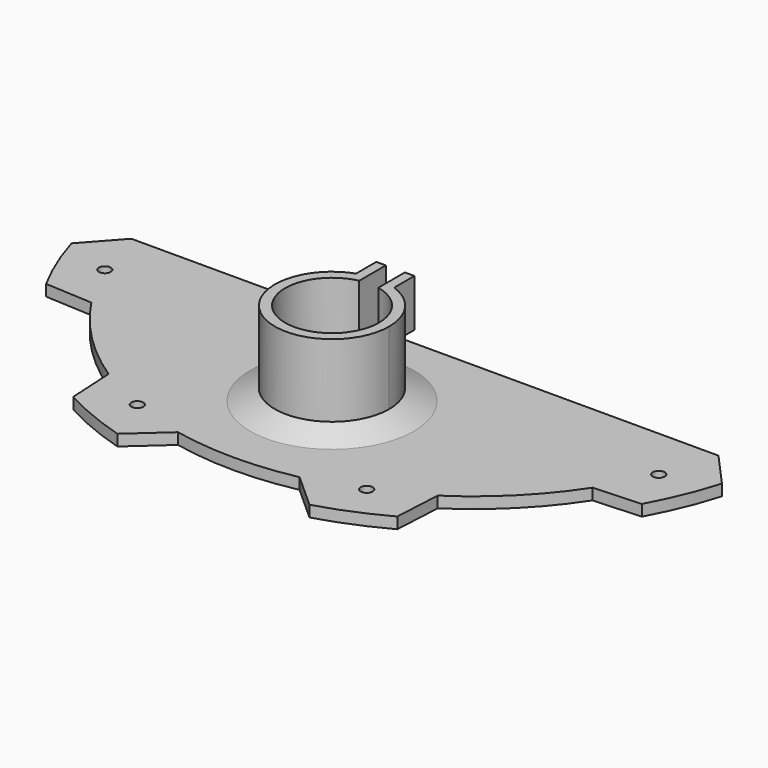
from build123d import *

# Parameters (mm, degrees)
F0_R     = 1.5875
F0_R_2   = 22.225
F1_DEPTH = 2.9972
F2_DEPTH = 25.4
F3_DEPTH = 25.4
F4_DEPTH = 12.7
F5_DEPTH = 2.9972
F6_DEPTH = 5.9944


# Not quite as in the source:
# - a fillet or chamfer that OpenCascade refuses, or shapes differently, is made with other operations: its cross-section is extruded or revolved along the edge and cut away or added


with BuildPart() as f1:
    # F0 (on Top) → F1 (new body)
    with BuildSketch(Plane.XY):
        with BuildLine():
            Line((-78.3343552322, -16.2264228234), (-86.7801633577, -25.6357348999))
            ThreePointArc((-86.7801633577, -25.6357348999), (-83.5995491981, -34.6280670861), (-79.4900439712, -43.2356399943))
            Line((-79.4900439712, -43.2356399943), (-66.8645673974, -43.9169401718))
            ThreePointArc((-66.8645673974, -43.9169401718), (-56.5666333066, -56.5666333066), (-43.9169401718, -66.8645673974))
            Line((-43.9169401718, -66.8645673974), (-43.2356399943, -79.4900439712))
            ThreePointArc((-43.2356399943, -79.4900439712), (-34.6280670861, -83.5995491981), (-25.6357348999, -86.7801633577))
            Line((-25.6357348999, -86.7801633577), (-16.2264228234, -78.3343552322))
            ThreePointArc((-16.2264228234, -78.3343552322), (0, -79.9973), (16.2264228234, -78.3343552322))
            Line((16.2264228234, -78.3343552322), (25.6357348999, -86.7801633577))
            ThreePointArc((25.6357348999, -86.7801633577), (34.6280670861, -83.5995491981), (43.2356399943, -79.4900439712))
            Line((43.2356399943, -79.4900439712), (43.9169401718, -66.8645673974))
            ThreePointArc((43.9169401718, -66.8645673974), (56.5666333066, -56.5666333066), (66.8645673974, -43.9169401718))
            Line((66.8645673974, -43.9169401718), (79.4900439712, -43.2356399943))
            ThreePointArc((79.4900439712, -43.2356399943), (83.5995491981, -34.6280670861), (86.7801633577, -25.6357348999))
            Line((86.7801633577, -25.6357348999), (78.3343552322, -16.2264228234))
            Line((78.3343552322, -16.2264228234), (-78.3343552322, -16.2264228234))
        make_face()
        with Locations((-30.6136413439, -73.9078681262)):
            Circle(F0_R, mode=Mode.SUBTRACT)
        with Locations((30.6136413439, -73.9078681262)):
            Circle(F0_R, mode=Mode.SUBTRACT)
        with Locations((0, -47.218952328)):
            Circle(F0_R_2, mode=Mode.SUBTRACT)
        with Locations((-73.9078681262, -30.6136413439)):
            Circle(F0_R, mode=Mode.SUBTRACT)
        with Locations((73.9078681262, -30.6136413439)):
            Circle(F0_R, mode=Mode.SUBTRACT)
        with Locations((0, -47.218952328)):
            Circle(F0_R_2)
        with BuildLine():
            ThreePointArc((5.08, -32.8505425343), (12.4434078933, -38.4201342255), (15.24, -47.218952328))
            ThreePointArc((15.24, -47.218952328), (-8.7988181024, -59.6623602213), (-5.08, -32.8505425343))
            Line((-5.08, -32.8505425343), (-5.08, -26.0933935642))
            Line((-5.08, -26.0933935642), (-2.54, -26.0933935642))
            Line((-2.54, -26.0933935642), (-2.54, -32.1921096789))
            ThreePointArc((-2.54, -32.1921096789), (0, -31.978952328), (2.54, -32.1921096789))
            Line((2.54, -32.1921096789), (2.54, -26.0933935642))
            Line((2.54, -26.0933935642), (5.08, -26.0933935642))
            Line((5.08, -26.0933935642), (5.08, -32.8505425343))
        make_face(mode=Mode.SUBTRACT)
        with BuildLine():
            ThreePointArc((-5.08, -32.8505425343), (-8.7988181024, -59.6623602213), (15.24, -47.218952328))
            ThreePointArc((15.24, -47.218952328), (12.4434078933, -38.4201342255), (5.08, -32.8505425343))
            ThreePointArc((5.08, -32.8505425343), (3.8241970996, -32.466558741), (2.54, -32.1921096789))
            Line((2.54, -32.1921096789), (2.54, -34.9700344064))
            ThreePointArc((2.54, -34.9700344064), (9.7021059634, -39.3223245588), (12.5095, -47.218952328))
            ThreePointArc((12.5095, -47.218952328), (-7.8966277692, -56.9210582914), (-2.54, -34.9700344064))
            Line((-2.54, -34.9700344064), (-2.54, -32.1921096789))
            ThreePointArc((-2.54, -32.1921096789), (-3.8241970996, -32.466558741), (-5.08, -32.8505425343))
        make_face()
        with BuildLine():
            ThreePointArc((2.54, -32.1921096789), (3.8241970996, -32.466558741), (5.08, -32.8505425343))
            Line((5.08, -32.8505425343), (5.08, -26.0933935642))
            Line((5.08, -26.0933935642), (2.54, -26.0933935642))
            Line((2.54, -26.0933935642), (2.54, -32.1921096789))
        make_face()
        with BuildLine():
            Line((-5.08, -26.0933935642), (-5.08, -32.8505425343))
            ThreePointArc((-5.08, -32.8505425343), (-3.8241970996, -32.466558741), (-2.54, -32.1921096789))
            Line((-2.54, -32.1921096789), (-2.54, -26.0933935642))
            Line((-2.54, -26.0933935642), (-5.08, -26.0933935642))
        make_face()
        with BuildLine():
            Line((2.54, -34.9700344064), (2.54, -32.1921096789))
            ThreePointArc((2.54, -32.1921096789), (0, -31.978952328), (-2.54, -32.1921096789))
            Line((-2.54, -32.1921096789), (-2.54, -34.9700344064))
            ThreePointArc((-2.54, -34.9700344064), (0, -34.709452328), (2.54, -34.9700344064))
        make_face()
        with BuildLine():
            ThreePointArc((12.5095, -47.218952328), (9.7021059634, -39.3223245588), (2.54, -34.9700344064))
            ThreePointArc((2.54, -34.9700344064), (0, -34.709452328), (-2.54, -34.9700344064))
            ThreePointArc((-2.54, -34.9700344064), (-7.8966277692, -56.9210582914), (12.5095, -47.218952328))
        make_face()
    extrude(amount=F1_DEPTH)

    # F0 (on Top) → F2 (join)
    with BuildSketch(Plane.XY):
        with BuildLine():
            ThreePointArc((-5.08, -32.8505425343), (-8.7988181024, -59.6623602213), (15.24, -47.218952328))
            ThreePointArc((15.24, -47.218952328), (12.4434078933, -38.4201342255), (5.08, -32.8505425343))
            ThreePointArc((5.08, -32.8505425343), (3.8241970996, -32.466558741), (2.54, -32.1921096789))
            Line((2.54, -32.1921096789), (2.54, -34.9700344064))
            ThreePointArc((2.54, -34.9700344064), (9.7021059634, -39.3223245588), (12.5095, -47.218952328))
            ThreePointArc((12.5095, -47.218952328), (-7.8966277692, -56.9210582914), (-2.54, -34.9700344064))
            Line((-2.54, -34.9700344064), (-2.54, -32.1921096789))
            ThreePointArc((-2.54, -32.1921096789), (-3.8241970996, -32.466558741), (-5.08, -32.8505425343))
        make_face()
    extrude(amount=F2_DEPTH)

    # F0 (on Top) → F3 (join)
    with BuildSketch(Plane.XY):
        with BuildLine():
            ThreePointArc((-5.08, -32.8505425343), (-8.7988181024, -59.6623602213), (15.24, -47.218952328))
            ThreePointArc((15.24, -47.218952328), (12.4434078933, -38.4201342255), (5.08, -32.8505425343))
            ThreePointArc((5.08, -32.8505425343), (3.8241970996, -32.466558741), (2.54, -32.1921096789))
            Line((2.54, -32.1921096789), (2.54, -34.9700344064))
            ThreePointArc((2.54, -34.9700344064), (9.7021059634, -39.3223245588), (12.5095, -47.218952328))
            ThreePointArc((12.5095, -47.218952328), (-7.8966277692, -56.9210582914), (-2.54, -34.9700344064))
            Line((-2.54, -34.9700344064), (-2.54, -32.1921096789))
            ThreePointArc((-2.54, -32.1921096789), (-3.8241970996, -32.466558741), (-5.08, -32.8505425343))
        make_face()
        with BuildLine():
            ThreePointArc((2.54, -32.1921096789), (3.8241970996, -32.466558741), (5.08, -32.8505425343))
            Line((5.08, -32.8505425343), (5.08, -26.0933935642))
            Line((5.08, -26.0933935642), (2.54, -26.0933935642))
            Line((2.54, -26.0933935642), (2.54, -32.1921096789))
        make_face()
        with BuildLine():
            Line((-5.08, -26.0933935642), (-5.08, -32.8505425343))
            ThreePointArc((-5.08, -32.8505425343), (-3.8241970996, -32.466558741), (-2.54, -32.1921096789))
            Line((-2.54, -32.1921096789), (-2.54, -26.0933935642))
            Line((-2.54, -26.0933935642), (-5.08, -26.0933935642))
        make_face()
    extrude(amount=F3_DEPTH)

    # F0 (on Top) → F4 (cut)
    with BuildSketch(Plane.XY):
        with BuildLine():
            ThreePointArc((2.54, -32.1921096789), (3.8241970996, -32.466558741), (5.08, -32.8505425343))
            Line((5.08, -32.8505425343), (5.08, -26.0933935642))
            Line((5.08, -26.0933935642), (2.54, -26.0933935642))
            Line((2.54, -26.0933935642), (2.54, -32.1921096789))
        make_face()
        with BuildLine():
            Line((-5.08, -26.0933935642), (-5.08, -32.8505425343))
            ThreePointArc((-5.08, -32.8505425343), (-3.8241970996, -32.466558741), (-2.54, -32.1921096789))
            Line((-2.54, -32.1921096789), (-2.54, -26.0933935642))
            Line((-2.54, -26.0933935642), (-5.08, -26.0933935642))
        make_face()
    extrude(amount=F4_DEPTH, mode=Mode.SUBTRACT)

    # F0 (on Top) → F5 (join)
    with BuildSketch(Plane.XY):
        with BuildLine():
            ThreePointArc((2.54, -32.1921096789), (3.8241970996, -32.466558741), (5.08, -32.8505425343))
            Line((5.08, -32.8505425343), (5.08, -26.0933935642))
            Line((5.08, -26.0933935642), (2.54, -26.0933935642))
            Line((2.54, -26.0933935642), (2.54, -32.1921096789))
        make_face()
        with BuildLine():
            Line((-5.08, -26.0933935642), (-5.08, -32.8505425343))
            ThreePointArc((-5.08, -32.8505425343), (-3.8241970996, -32.466558741), (-2.54, -32.1921096789))
            Line((-2.54, -32.1921096789), (-2.54, -26.0933935642))
            Line((-2.54, -26.0933935642), (-5.08, -26.0933935642))
        make_face()
    extrude(amount=F5_DEPTH)

    # F0 (on Top) → F6 (join)
    with BuildSketch(Plane.XY):
        with Locations((0, -47.218952328)):
            Circle(F0_R_2)
        with BuildLine():
            ThreePointArc((5.08, -32.8505425343), (12.4434078933, -38.4201342255), (15.24, -47.218952328))
            ThreePointArc((15.24, -47.218952328), (-8.7988181024, -59.6623602213), (-5.08, -32.8505425343))
            Line((-5.08, -32.8505425343), (-5.08, -26.0933935642))
            Line((-5.08, -26.0933935642), (-2.54, -26.0933935642))
            Line((-2.54, -26.0933935642), (-2.54, -32.1921096789))
            ThreePointArc((-2.54, -32.1921096789), (0, -31.978952328), (2.54, -32.1921096789))
            Line((2.54, -32.1921096789), (2.54, -26.0933935642))
            Line((2.54, -26.0933935642), (5.08, -26.0933935642))
            Line((5.08, -26.0933935642), (5.08, -32.8505425343))
        make_face(mode=Mode.SUBTRACT)
        with BuildLine():
            ThreePointArc((2.54, -32.1921096789), (3.8241970996, -32.466558741), (5.08, -32.8505425343))
            Line((5.08, -32.8505425343), (5.08, -26.0933935642))
            Line((5.08, -26.0933935642), (2.54, -26.0933935642))
            Line((2.54, -26.0933935642), (2.54, -32.1921096789))
        make_face()
        with BuildLine():
            Line((-5.08, -26.0933935642), (-5.08, -32.8505425343))
            ThreePointArc((-5.08, -32.8505425343), (-3.8241970996, -32.466558741), (-2.54, -32.1921096789))
            Line((-2.54, -32.1921096789), (-2.54, -26.0933935642))
            Line((-2.54, -26.0933935642), (-5.08, -26.0933935642))
        make_face()
    extrude(amount=F6_DEPTH)

    # F7: chamfer of 6.858 x 3.1496 on 1 edges, made by hand


with BuildPart() as f7_tool2:
    # F7_s3 → F7_t4 (revolve)
    with BuildSketch(Plane.XZ.offset(47.218952328)):
        Polygon((22.225, 2.8448), (15.367, 5.9944), (22.225, 5.9944), align=None)
    revolve(axis=Axis((0, -47.218952328, 5.9944), (0, 0, 1)))

    split(bisect_by=Plane.XY.offset(2.9972), keep=Keep.TOP)


with BuildPart() as f1_1:
    add(f1.part)

    # F7_t1: cut F7_tool2
    add(f7_tool2.part, mode=Mode.SUBTRACT)


solid = f1_1.part
